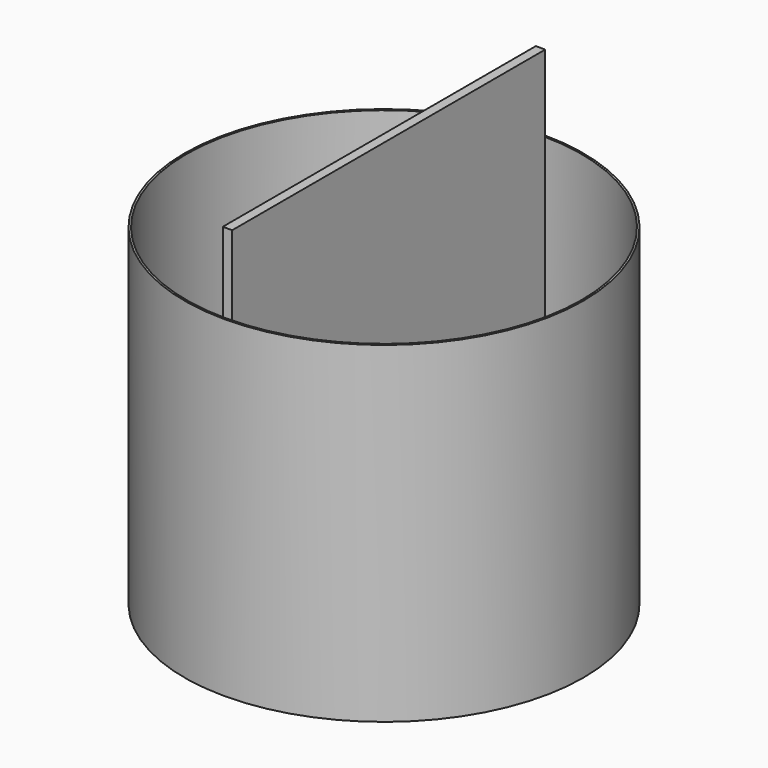
from build123d import *

# Parameters (mm, degrees)
F0_R     = 250
F1_DEPTH = 24
F2_W     = 12
F2_H     = 500
F3_DEPTH = 524
F6_R     = 255
F6_R_2   = 252.5
F7_DEPTH = 424


# Not quite as in the source:
# - the program builds the solid bodies; features that only make, move or delete a surface that nothing else refers to are left out


with BuildPart() as f1:
    # F0 (on Top) → F1 (new body)
    with BuildSketch(Plane.XY):
        Circle(F0_R)
    extrude(amount=F1_DEPTH)

    # F2 (on Top) → F3 (join)
    with BuildSketch(Plane.XY):
        Rectangle(F2_W, F2_H)
    extrude(amount=F3_DEPTH)


with BuildPart() as f7:
    # F6 (on Top) → F7 (new body)
    with BuildSketch(Plane.XY):
        Circle(F6_R)
        Circle(F6_R_2, mode=Mode.SUBTRACT)
    extrude(amount=F7_DEPTH)


solid = Compound([f1.part, f7.part])
